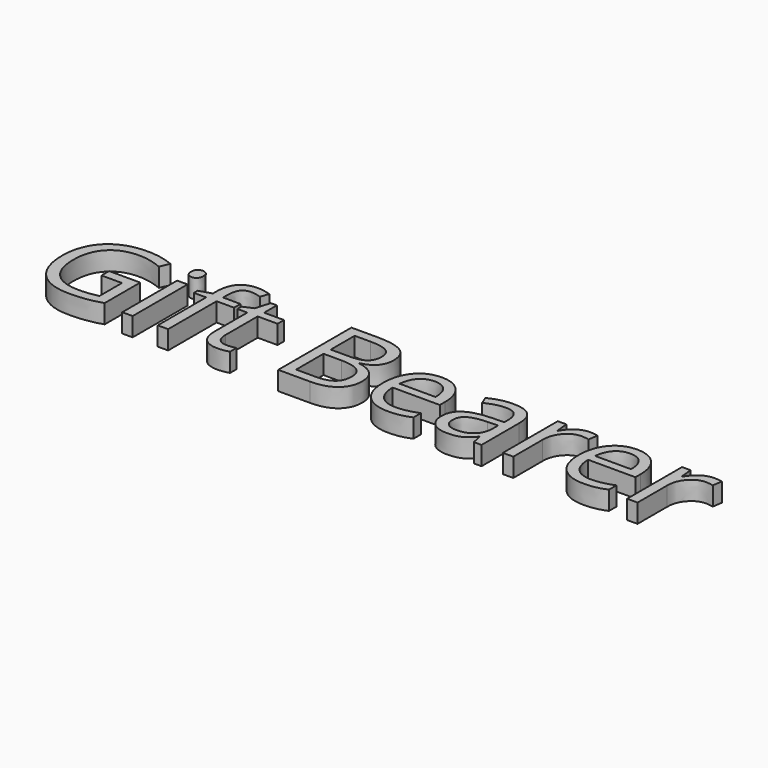
from build123d import *

# Parameters (mm, degrees)
F0_TEXT_SIZE = 17.3426402902
F1_DEPTH     = 2.54


# Not quite as in the source:
# - Text() gives the source's letters only with a copy of the font that has no kerning and outlines rounded to 1/6400 em; it was checked with that copy


with BuildPart() as f1:
    # F0 (on Top) → F1 (new body)
    with BuildSketch(Plane.XY):
        with Locations((0, 12.8066494955)):
            Text('Gift Bearer', F0_TEXT_SIZE, font='Open Sans', text_align=(TextAlign.LEFT, TextAlign.BOTTOM))
    extrude(amount=F1_DEPTH)


solid = f1.part
